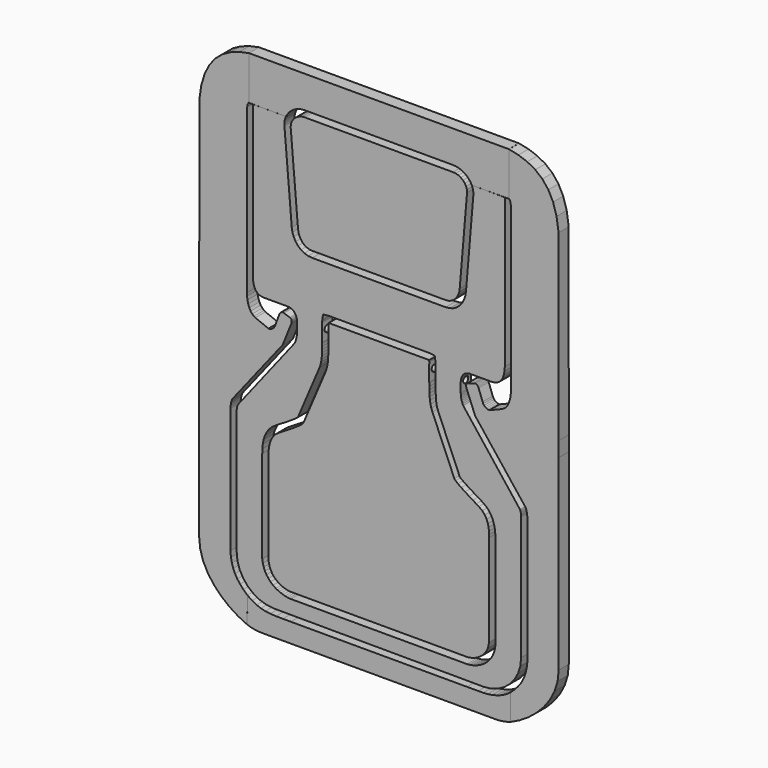
from build123d import *

# Parameters (mm, degrees)
F1_DEPTH = 20
F2_R     = 5
F3_DEPTH = 138
F7_R     = 4.8289387716
F8_DEPTH = 20
F6_R     = 4.8289387716


with BuildPart() as f1:
    # F0 (on Front) → F1 (new body)
    with BuildSketch(Plane.XZ):
        Polygon((-236.2401408257, -220.8566135145), (-235.9931658525, -22.8898533906), (-235.9213222059, -20.8247963317), (-235.7645000634, -18.8341700867), (-235.5214058411, -16.9189697199), (-235.1910444748, -15.080488815), (-234.771724355, -13.3195234235), (-234.2625499238, -11.637367129), (-233.6621280911, -10.0351145023), (-232.9691652733, -8.5136611013), (-153.5204408774, 92.5275618029), (-139.7851695402, 126.6684188842), (-139.421274505, 128.1299694109), (-139.2460436719, 129.4539025371), (-139.2637558174, 130.6369345504), (-139.4793862635, 131.6759807514), (-139.8974127996, 132.5673594018), (-140.5224127218, 133.3078862959), (-141.3589633263, 133.8939792018), (-142.4115424025, 134.3226529265), (-151.617877828, 137.2894373052), (-152.7547388552, 137.5879566121), (-153.8255276091, 137.6534318468), (-154.8304431027, 137.4865595542), (-155.7697838551, 137.0881357859), (-156.6436493729, 136.4588570869), (-157.4522386689, 135.5995195087), (-158.195750756, 134.5106205835), (-158.8743846471, 133.1930558692), (-165.3383227063, 115.810276627), (-166.2609463776, 113.5963579405), (-167.5404001271, 111.6587686257), (-169.1666338047, 110.0537298188), (-171.1294977542, 108.8378606817), (-173.4192403447, 108.0669843248), (-176.0257119199, 107.7976204035), (-196.7799682144, 116.1239209122), (-198.8963705941, 117.5921383701), (-201.7156864351, 119.6827685829), (-204.219765888, 122.8738404674), (-206.3468154562, 126.9251454881), (-208.034743124, 131.5967736286), (-209.2216558883, 136.6485163532), (-209.8457602527, 141.8405631521), (-209.8449642012, 146.9326059831), (-209.7976986443, 404.8079122297), (-208.915972118, 409.1425120727), (-207.8829958097, 411.038408191), (-207.0924171785, 411.9953615825), (-206.8530046943, 480.9579982842), (-221.869321884, 477.7549856273), (-235.8005213931, 472.8562838007), (-248.4462967665, 465.9490445707), (-259.6062420429, 456.7204197036), (-269.0801502739, 444.8572624465), (-276.6678145108, 430.0467245657), (-282.1688287923, 411.9759578276), (-285.3828866635, 390.3319149856), (-285.4361226066, 100.890281667), (-285.4405008898, 77.3006889954), (-285.4949309101, -218.1556108255), (-283.82521292, -234.2816237854), (-279.0882090513, -249.5766585014), (-271.7011497886, -263.8817036891), (-262.0811661102, -277.0380465838), (-250.6454885006, -288.8868749142), (-237.8112479381, -299.2693764089), (-223.9957744137, -308.0267387968), (-209.6160993992, -315.0000503001), (-209.4870715937, -273.9394860296), (-215.614645859, -268.17699849), (-220.8586350172, -262.4428406297), (-225.2580135498, -256.6031064413), (-228.8599475071, -250.5158997474), (-231.7118019526, -244.0394238772), (-233.8609419496, -237.0318821601), (-235.354633055, -229.3515774316), align=None)
    extrude(amount=F1_DEPTH)


with BuildPart() as f1b:
    # F0 (on Front) → F1, piece 2 (new body)
    with BuildSketch(Plane.XZ):
        Polygon((204.0437958057, 480.9392354422), (204.0437958057, 455.6201073027), (204.1952446081, 411.9953615825), (204.9858232393, 411.038408191), (206.0187995476, 409.1425120727), (206.9005260739, 404.8079122297), (206.9477916308, 146.9326059831), (206.9485876823, 141.8405631521), (206.3244833179, 136.6485163532), (205.1375705536, 131.5967736286), (203.4496428858, 126.9251454881), (201.3225933176, 122.8738404674), (198.8185138647, 119.6827685829), (195.9991980237, 117.5921383701), (193.882795644, 116.1239209122), (173.1285393495, 107.7976204035), (170.5220677743, 108.0669843248), (168.2323251838, 108.8378606817), (166.2694612344, 110.0537298188), (164.6432275567, 111.6587686257), (163.3637738072, 113.5963579405), (162.4411501359, 115.810276627), (155.9772120767, 133.1930558692), (155.2985781856, 134.5106205835), (154.5550660985, 135.5995195087), (153.7464768025, 136.4588570869), (152.8726112847, 137.0881357859), (151.9332705323, 137.4865595542), (150.9283550387, 137.6534318468), (149.8575662848, 137.5879566121), (148.7207052576, 137.2894373052), (139.5143698321, 134.3226529265), (138.4617907559, 133.8939792018), (137.6252401514, 133.3078862959), (137.0002402292, 132.5673594018), (136.5822136931, 131.6759807514), (136.366583247, 130.6369345504), (136.3488711015, 129.4539025371), (136.5241019346, 128.1299694109), (136.8879969698, 126.6684188842), (150.623268307, 92.5275618029), (230.0719927029, -8.5136611013), (230.7649555208, -10.0351145023), (231.3653773534, -11.637367129), (231.8745517846, -13.3195234235), (232.2938719044, -15.080488815), (232.6242332707, -16.9189697199), (232.867327493, -18.8341700867), (233.0241496355, -20.8247963317), (233.0959932821, -22.8898533906), (233.3429682553, -220.8566135145), (232.4574604846, -229.3515774316), (230.9637693792, -237.0318821601), (228.8146293822, -244.0394238772), (225.9627749367, -250.5158997474), (222.3608409794, -256.6031064413), (217.9614624468, -262.4428406297), (212.7174732886, -268.17699849), (206.5815084412, -273.9473766928), (206.7189268288, -315.0000503001), (221.0986018433, -308.0267387968), (234.9140753677, -299.2693764089), (247.7483159302, -288.8868749142), (259.1839935398, -277.0380465838), (268.8039772183, -263.8817036891), (276.1910364809, -249.5766585014), (280.9280403496, -234.2816237854), (282.5977583397, -218.1556108255), (282.5433283194, 77.3006889954), (282.5389500362, 100.890281667), (282.4857140931, 390.3319149856), (279.2716562219, 411.9759578276), (273.7706419404, 430.0467245657), (266.1829777035, 444.8572624465), (256.7090694725, 456.7204197036), (245.5491241961, 465.9490445707), (232.9033488227, 472.8562838007), (218.9721493136, 477.7549856273), align=None)
    extrude(amount=F1_DEPTH)


with BuildPart() as f1c:
    # F0 (on Front) → F1, piece 3 (new body)
    with BuildSketch(Plane.XZ):
        Polygon((203.955832124, 480.9579982842), (-206.8530046943, 480.9579982842), (-206.8530046943, 411.8710780444), (-148.32779704, 411.8710780444), (-146.1237294905, 415.7605856007), (-143.3535698287, 419.2941586368), (-140.0862760144, 422.4217454154), (-136.3906069947, 425.0931946931), (-132.3354212231, 427.2582557197), (-127.9894776464, 428.8667772519), (-123.4216347183, 429.8687075523), (-118.7006513858, 430.2137958712), (115.5793903223, 430.2137958712), (120.3002741484, 429.8687075523), (124.8681170765, 428.8667772519), (129.2141601596, 427.2582557197), (133.2693459313, 425.0931946931), (136.965014951, 422.4217454154), (140.2323087652, 419.2941586368), (143.002468427, 415.7605856007), (145.2065359765, 411.8710780444), (204.043795813, 411.8710780444), (204.0437958057, 455.6201073027), align=None)
    extrude(amount=F1_DEPTH)


with BuildPart() as f1d:
    # F0 (on Front) → F1, piece 4 (new body)
    with BuildSketch(Plane.XZ):
        Polygon((223.2277879737, -220.2793986993), (223.2201287769, -24.1411222171), (223.1834109021, -22.9348056978), (223.1053978566, -21.7009258958), (222.9788256705, -20.4528166736), (222.7965298804, -19.2040109063), (222.5513460229, -17.9679419628), (222.2360101284, -16.7581427183), (221.8433577334, -15.5878475287), (221.3662243745, -14.4706887757), (131.7147568873, 100.6557449982), (131.5753483709, 100.9489904641), (130.751932616, 102.8088652526), (130.0341926957, 104.697696414), (129.4197404556, 106.6138918451), (128.9062872477, 108.5557599366), (128.491544424, 110.521808092), (128.1731238299, 112.510145689), (127.9487368175, 114.5191806246), (127.8160947388, 116.5474203023), (127.8069401468, 116.7610606196), (127.8069401468, 132.1765976291), (127.8092287948, 132.2837660603), (128.1133204621, 135.5273773429), (128.8769328492, 138.5635177071), (130.0914088962, 141.3206420259), (131.7484895689, 143.727702704), (133.8395178075, 145.7132541208), (136.3562345777, 147.2060496683), (139.2900823262, 148.1348427386), (142.6327025122, 148.4281877108), (151.9998403377, 148.427988698), (176.0318386222, 148.4266951143), (181.0540279354, 148.9439295668), (185.3838514695, 150.3379152236), (189.0327524644, 152.5945221711), (192.0121741604, 155.6992224695), (194.3333607846, 159.6374881793), (196.0077555771, 164.3951893866), (197.0466027652, 169.9577981518), (197.4614450954, 176.3109855482), (197.4614450954, 410.7804875098), (197.4383596023, 410.9938293078), (197.3725858484, 411.1956283593), (197.2692981682, 411.3804118103), (197.134114194, 411.5427714329), (197.1443950076, 411.5569647622), (196.5979305721, 411.7211087847), (196.3712392069, 411.743877759), (145.2126502991, 411.8552207947), (145.893727421, 410.2789750742), (146.4817109492, 408.6438853237), (146.9664067972, 406.9687939861), (147.3437352012, 405.2564872416), (147.6096163972, 403.5100497897), (147.7602691408, 401.7321683041), (147.7914146551, 399.9259274843), (147.6990726829, 398.0941135106), (136.1148319649, 260.6629890668), (135.0332965159, 254.2288034318), (132.9544080625, 248.217918174), (129.9578712596, 242.7642689558), (126.1231917493, 238.0018909461), (121.5299746801, 234.0647198071), (116.2578252005, 231.0865916948), (110.3863484591, 229.2014422716), (103.9951496043, 228.5433067062), (-107.1165101742, 228.5433067062), (-113.507709029, 229.2014422715), (-119.3791857704, 231.0864921883), (-124.65133525, 234.0646203006), (-129.2445523192, 238.0018909461), (-133.0792318295, 242.7641694494), (-136.0757686324, 248.2178186676), (-138.1546570858, 254.2287039253), (-139.2361925347, 260.6629890668), (-150.8203337463, 398.0941135106), (-150.9126757186, 399.9259274843), (-150.8815302042, 401.7321683041), (-150.7308774607, 403.5100497897), (-150.4649962646, 405.2565867481), (-150.0876678607, 406.9687939861), (-149.6029720127, 408.6438853237), (-149.0149884845, 410.2789750742), (-148.3398526907, 411.8315279484), (-199.4782537222, 411.8200540543), (-199.6872723103, 411.8174314499), (-199.8887482767, 411.7822187974), (-200.0736312341, 411.6789311172), (-200.2364237628, 411.5433038454), (-200.3720510346, 411.3805113167), (-200.4753387148, 411.1956283593), (-200.5411124688, 410.9938293078), (-200.5641979618, 410.7803880034), (-200.5668846356, 382.1922885502), (-200.5737505797, 352.6668384732), (-200.582507146, 322.5165874869), (-200.5911642059, 292.0537867862), (-200.5977316306, 261.591085592), (-200.6001197851, 231.4407350992), (-200.5961395277, 201.9152850223), (-200.5838007297, 173.3270860626), (-200.3715535024, 167.7074601098), (-199.6535150628, 162.7834836486), (-198.4225209475, 158.5645102838), (-196.6720037317, 155.0601921399), (-194.3948984585, 152.2797833152), (-191.5843391839, 150.2328364276), (-188.2334599636, 148.928904095), (-184.3353948538, 148.3773399222), (-155.1025932041, 148.427988698), (-145.7354553786, 148.4281877108), (-142.3928351926, 148.1348427386), (-139.4589874441, 147.2060496683), (-136.9422706739, 145.7132541208), (-134.8512424354, 143.727702704), (-133.1941617626, 141.3206420259), (-131.9796857156, 138.5635177071), (-131.2160733285, 135.5273773429), (-130.9119816612, 132.2837660603), (-130.9096930132, 132.1765976291), (-130.9096930132, 116.7610606196), (-130.9188476053, 116.5474203023), (-131.051489684, 114.5191806246), (-131.2758766963, 112.510145689), (-131.5942972904, 110.521808092), (-132.0090401141, 108.5557599366), (-132.5224933221, 106.6138918451), (-133.1369455621, 104.697696414), (-133.8546854824, 102.8088652526), (-134.6781012373, 100.9489904641), (-134.8175097537, 100.6557449982), (-224.4061389543, -13.8424297428), (-224.8832723132, -14.9595884957), (-225.2759247082, -16.1298836853), (-225.5912606027, -17.3396829298), (-225.8364444602, -18.5757518733), (-226.0187402503, -19.8245576406), (-226.1453124364, -21.0726668629), (-226.2233254819, -22.3065466648), (-226.2600433567, -23.5128631841), (-226.2600433567, -219.1687853532), (-225.0406914943, -231.1563256548), (-221.5462244875, -242.3423416174), (-216.0224232322, -252.4811518513), (-208.7146705987, -261.3272739798), (-199.8685484703, -268.6350266132), (-189.7297382364, -274.1588278685), (-178.5437222738, -277.6532948754), (-166.5561819721, -278.8726467377), (163.5239265892, -279.9832600838), (175.5114668909, -278.7639082215), (186.6974828534, -275.2694412146), (196.8362930873, -269.7455404529), (205.6823157094, -262.4377878194), (212.9900683428, -253.5917651974), (218.5139691046, -243.4529549635), (222.0084361114, -232.2669390009), align=None)
        Polygon((159.172562738, -21.7430417198), (161.4852913152, -23.1856860237), (167.3904012318, -27.3160986607), (172.1425300787, -32.0750934517), (175.8544186475, -37.385552909), (178.6387082231, -43.1699615192), (180.6081395973, -49.3511022884), (181.8753540552, -55.8515592095), (182.5529928819, -62.5940157821), (182.7538963755, -69.5012550121), (182.7538963755, -215.6948166721), (182.6949885656, -216.2338430339), (181.8325662879, -221.5304710967), (180.4359934637, -226.5561431351), (178.512136037, -231.2906593429), (176.0678599519, -235.7141184329), (173.109931646, -239.8061215858), (169.6452170635, -243.5466680079), (165.6804826418, -246.915557893), (161.2226938315, -249.8926909409), (158.6913496152, -251.2778205251), (155.9229810693, -252.5872257117), (152.9787846515, -253.7873728319), (149.9195587942, -254.8446287106), (146.8064004487, -255.7253601725), (143.7003070602, -256.3961330551), (140.6623755801, -256.8231151705), (137.753503947, -256.9729718625), (-140.8603365773, -256.9729718625), (-143.7697057425, -256.8232146769), (-146.8081347548, -256.3962325616), (-149.9145266627, -255.7255591853), (-153.0279835275, -254.8449272299), (-156.0875079041, -253.7877708577), (-159.0321023476, -252.5876237374), (-161.8008689193, -251.2782185508), (-164.3327106677, -249.8928899538), (-168.7906984909, -246.9157569059), (-172.7556319254, -243.5469665273), (-176.2204460145, -239.8064201051), (-179.1784738268, -235.7144169522), (-181.6228494183, -231.2909578622), (-183.546706845, -226.556342148), (-184.9433791756, -221.5305706031), (-185.8058014533, -216.2338430339), (-185.8647092632, -215.6948166721), (-185.8647092632, -69.5012550121), (-185.6638057697, -62.5940157821), (-184.9861669429, -55.8515592095), (-183.7189524851, -49.3511022884), (-181.7495211108, -43.1699615192), (-178.9652315352, -37.385552909), (-175.2533429665, -32.0750934517), (-170.5012141196, -27.3160986607), (-164.5961042029, -23.1856860237), (-162.2833756257, -21.7430417198), (-159.96139295, -20.3135322654), (-157.6331413689, -18.8928788837), (-155.3013075561, -17.4769023046), (-152.9688767047, -16.0613237511), (-150.6387345013, -14.6417649403), (-148.3137666325, -13.2142456146), (-145.9968587851, -11.7743874909), (-144.5811807252, -10.8856955141), (-143.166796249, -9.9917296963), (-141.755197953, -9.0913954667), (-140.3476794209, -8.1836977607), (-138.9458327555, -7.2673429949), (-137.5511505536, -6.3413361049), (-136.1648268923, -5.4046820262), (-134.7885533809, -4.4561866816), (-134.2185805176, -4.0609471193), (-133.5732812824, -3.6130686525), (-132.8776317909, -3.1242930406), (-132.1565086518, -2.6065610559), (-131.4348879805, -2.0716144579), (-130.7378453988, -1.5313940188), (-130.0901580092, -0.9976414981), (-129.5169014335, -0.4823971743), (-95.3820147384, 79.6976000171), (-93.8836468305, 83.8717954858), (-92.8265899647, 88.169677454), (-92.1287513315, 92.5605979395), (-91.7079386152, 97.0141079731), (-91.4820590063, 101.4997585853), (-91.3690196954, 105.9869017941), (-91.2866283667, 110.4449891237), (-91.1527922108, 114.8435716048), (-91.1071187568, 115.9087879983), (-91.1071187568, 132.581787835), (-91.1292091855, 143.6654116753), (-91.1276170826, 144.1858303337), (-91.1202536063, 144.7091346787), (-91.1059246796, 145.2340311268), (-91.0837347444, 145.7594251069), (-91.0525892301, 146.2843215549), (-91.0114930722, 146.8075263935), (-90.9595507128, 147.3278455455), (-90.8955680746, 147.8441844401), (-89.8340334192, 155.613447922), (-82.0319328135, 156.3977576477), (-81.4267346719, 156.4495009943), (-80.8193473888, 156.4844277532), (-80.2110645477, 156.5041300274), (-79.603776771, 156.5103989329), (76.4929638833, 156.5103989329), (77.10025166, 156.5041300274), (77.7085345011, 156.4844277532), (78.3159217842, 156.4495009943), (78.9211199258, 156.3977576477), (86.7232205315, 155.613447922), (87.7847551869, 147.8441844401), (87.8487378251, 147.3278455455), (87.9006801845, 146.8075263935), (87.9417763424, 146.2843215549), (87.9729218567, 145.7594251069), (87.9951117919, 145.2340311268), (88.0094407186, 144.7091346787), (88.0168041948, 144.1858303337), (88.0183962978, 143.6654116753), (87.9963058691, 132.6015896157), (87.9963058691, 115.9087879983), (88.0419793231, 114.8435716048), (88.175815479, 110.4449891237), (88.2582068077, 105.9869017941), (88.3712461186, 101.4997585853), (88.5971257275, 97.0141079731), (89.0179384438, 92.5605979395), (89.715777077, 88.169677454), (90.7728339428, 83.8717954858), (92.2712018507, 79.6976000171), (126.4060885458, -0.4823971743), (126.9793451215, -0.9976414981), (127.6270325111, -1.5313940188), (128.3240750928, -2.0716144579), (129.0456957641, -2.6065610559), (129.7668189031, -3.1242930406), (130.4624683947, -3.6130686525), (131.1077676298, -4.0609471193), (131.6777404932, -4.4561866816), (133.0540140045, -5.4046820262), (134.4403376659, -6.3413361049), (135.8350198678, -7.2673429949), (137.2368665331, -8.1836977607), (138.6443850653, -9.0913954667), (140.0559833613, -9.9917296963), (141.4703678375, -10.8856955141), (142.8860458973, -11.7743874909), (145.2029537448, -13.2142456146), (147.5279216136, -14.6417649403), (149.858063817, -16.0613237511), (152.1904946684, -17.4769023046), (154.5223284812, -18.8928788837), (156.8505800623, -20.3135322654), align=None, mode=Mode.SUBTRACT)
    extrude(amount=F1_DEPTH)


with BuildPart() as f1e:
    # F0 (on Front) → F1, piece 5 (new body)
    with BuildSketch(Plane.XZ):
        Polygon((-209.4869400458, -273.897623475), (-209.4870715937, -273.9394860296), (-209.4786810116, -273.9473766928), (-209.6160993992, -315.0000503001), (-206.6249359438, -315.9798901719), (-203.5794419746, -316.816142257), (-200.4831997232, -317.5127868129), (-197.3396919149, -318.0739036035), (-194.1525007813, -318.5034728862), (-190.9251090477, -318.8052759055), (-187.6612979587, -318.9834919317), (-184.3643512266, -319.0420017158), (181.3463778434, -319.0420017158), (184.6522801547, -318.9839894639), (187.9274349773, -318.8070670213), (191.1674640282, -318.5066570921), (194.3679890242, -318.078580406), (197.524631682, -317.5182596669), (200.6329142121, -316.8213165916), (203.6885578378, -315.9833728971), (206.6871842758, -315.0000503001), (206.5580249224, -273.897623475), (201.4267765557, -277.6289157986), (195.9224785618, -280.7933199584), (190.0532904684, -283.4033737653), (183.8274713096, -285.4716150301), (177.2534791326, -287.0106810702), (170.3394734649, -288.0331096964), (163.0937133409, -288.5515382261), (155.5244577945, -288.5785044701), (137.7999734524, -288.6133317226), (-140.8179468357, -288.6133317226), (-153.5557656621, -288.6107445553), (-164.197083396, -288.4730276483), (-173.1966444482, -288.0053474008), (-181.0092927361, -287.0128702117), (-188.0897726706, -285.3006629737), (-194.8930276753, -282.6739915921), (-201.8738021613, -278.9379229595), align=None)
    extrude(amount=F1_DEPTH)


with BuildPart() as f1f:
    # F0 (on Front) → F1, piece 6 (new body)
    with BuildSketch(Plane.XZ):
        Polygon((115.5793903223, 420.2631523071), (-118.7006513858, 420.2631523071), (-122.9420136985, 419.84263811), (-127.0822774727, 418.6307492304), (-130.9626304369, 416.7025135205), (-134.4240613072, 414.1323617944), (-137.3078573185, 410.9953219043), (-139.4552061996, 407.3660236772), (-140.7070966664, 403.3192959526), (-140.904815954, 398.9298680636), (-129.3206747424, 261.4987436197), (-128.5993525905, 257.0598610322), (-127.2190988217, 252.8343202427), (-125.2158352594, 248.9386432874), (-122.6257822461, 245.489750228), (-119.4847620986, 242.6040635945), (-115.8288956532, 240.3985034485), (-111.694104733, 238.9894923198), (-107.1165101742, 238.4939502703), (103.9951496043, 238.4939502703), (108.5727441631, 238.9894923198), (112.7074355769, 240.3985034485), (116.3633020223, 242.6040635945), (119.5043221698, 245.489750228), (122.0944746895, 248.9387427938), (124.0976387454, 252.8343202427), (125.4779920206, 257.0598610322), (126.1993141725, 261.4987436197), (137.7835548906, 398.9298680636), (137.5858356029, 403.3192959526), (136.3338456297, 407.3660236772), (134.186596255, 410.9953219043), (131.3028002437, 414.1323617944), (127.8412698671, 416.7024140141), (123.9610164092, 418.6307492304), (119.8207526351, 419.84263811), align=None)
    extrude(amount=F1_DEPTH)


with BuildPart() as f1g:
    # F0 (on Front) → F1, piece 7 (new body)
    with BuildSketch(Plane.XZ):
        Polygon((-140.8603365773, -247.0223282985), (137.753503947, -247.0223282985), (140.673321288, -246.7723681321), (145.0676249923, -245.8808899752), (150.4080358868, -244.1352485748), (156.1658762787, -241.3227986778), (161.8128665013, -237.2308950314), (166.8203288621, -231.646991889), (170.6599836941, -224.3583444911), (172.8032528114, -215.1525065978), (172.8032528114, -69.5012550121), (172.7594699797, -65.4569154419), (172.5060270881, -60.7872774301), (171.8602303208, -55.70777241), (170.6389878362, -50.433931321), (168.659506312, -45.1813846093), (165.7388929195, -40.1655637079), (161.69425483, -35.602099063), (156.3426992148, -31.7064221076), (152.276965761, -29.201248084), (146.9276987938, -25.9484822093), (140.8278547826, -22.2117170317), (134.510489703, -18.2548436184), (128.5086595309, -14.3413550111), (123.3554202419, -10.735142277), (119.5838278118, -7.6997979642), (117.7269382163, -5.4990141272), (83.1157142138, 75.7998334266), (81.3356435866, 80.7083863904), (80.0730064248, 85.6807229793), (79.2335701337, 90.6732593747), (78.7236991575, 95.6425112642), (78.4493599144, 100.5450938418), (78.3166183293, 105.3373237823), (78.2316398332, 109.9759157861), (78.1004903511, 114.4171865281), (78.045662305, 115.6954462003), (78.045662305, 132.6015896157), (78.0677527337, 143.685213456), (78.0642700085, 144.2466287659), (78.0458613179, 144.9623785575), (78.0027750313, 145.7426085193), (77.9257570501, 146.4970663143), (76.4929638833, 146.5597553688), (-79.603776771, 146.5597553688), (-81.0365699378, 146.4970663143), (-81.113587919, 145.7426085193), (-81.1566742056, 144.9623785575), (-81.1750828962, 144.2466287659), (-81.1785656214, 143.685213456), (-81.1564751927, 132.6015896157), (-81.1564751927, 115.6954462003), (-81.2113032388, 114.4171865281), (-81.3424527209, 109.9759157861), (-81.427431217, 105.3373237823), (-81.5601728021, 100.5450938418), (-81.8345120452, 95.6425112642), (-82.3443830214, 90.6732593747), (-83.1838193125, 85.6807229793), (-84.4464564743, 80.7083863904), (-86.2265271015, 75.7998334266), (-120.837751104, -5.4990141272), (-122.6946406995, -7.6997979642), (-126.4662331296, -10.735142277), (-131.6194724186, -14.3413550111), (-137.6213025907, -18.2548436184), (-143.9386676703, -22.2117170317), (-150.0385116815, -25.9484822093), (-155.3877786487, -29.201248084), (-159.4535121025, -31.7064221076), (-164.8050677177, -35.602099063), (-168.8497058072, -40.1655637079), (-171.7703191997, -45.1813846093), (-173.7498007239, -50.433931321), (-174.9710432085, -55.70777241), (-175.6168399759, -60.7872774301), (-175.8702828674, -65.4569154419), (-175.9140656991, -69.5012550121), (-175.9140656991, -215.1525065978), (-173.7707965818, -224.3583444911), (-169.9311417498, -231.646991889), (-164.9233808697, -237.2308950314), (-159.2761916342, -241.3227986778), (-153.5178537101, -244.1352485748), (-148.1767462706, -245.8808899752), (-143.781447502, -246.7723681321), align=None)
    extrude(amount=F1_DEPTH)


with BuildPart() as f3_tool:
    # F2 (on Right) → F3 (new body, symmetric)
    with BuildSketch(Plane.YZ):
        with Locations((-10.2011198178, 131.7112743855)):
            Circle(F2_R)
    extrude(amount=F3_DEPTH, both=True)


with BuildPart() as f1d_1:
    add(f1d.part)

    # F3: cut by f3_tool
    add(f3_tool.part, mode=Mode.SUBTRACT)


with BuildPart() as f1g_1:
    add(f1g.part)

    # F3: cut by f3_tool
    add(f3_tool.part, mode=Mode.SUBTRACT)


with BuildPart() as f8:
    # F7 (on offset) → F8 (new body, symmetric)
    with BuildSketch(Plane.YZ.offset(-87)):
        with Locations((-10.2011198178, 131.7112743855)):
            Circle(F7_R)
    extrude(amount=F8_DEPTH, both=True)


with BuildPart() as f8b:
    # F6 (on offset) → F8, piece 2 (new body, symmetric)
    with BuildSketch(Plane.YZ.offset(84)):
        with Locations((-10.2011198178, 131.7112743855)):
            Circle(F6_R)
    extrude(amount=F8_DEPTH, both=True)


solid = Compound([f1.part, f1b.part, f1c.part, f1e.part, f1f.part, f1d_1.part, f1g_1.part, f8.part, f8b.part])
